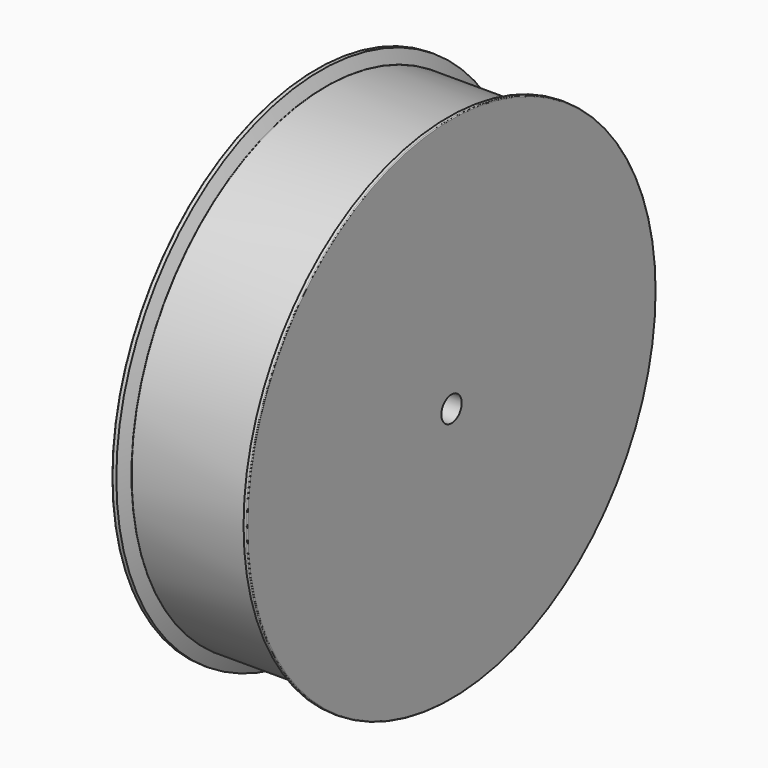
from build123d import *

# Parameters (mm, degrees)
F2_R     = 12.7
F3_DEPTH = 134.8161187441


# Not quite as in the source:
# - a feature names something its author has since deleted; it is built from what else it names


with BuildPart() as f1:
    # F0 (on Top) → F1 (revolve)
    with BuildSketch(Plane.XY):
        with BuildLine():
            Line((-3.6245174784, 29.0860664694), (-3.6245174784, 20.4818164694))
            Line((-3.6245174784, 20.4818164694), (-1.6004623353, 20.4818164694))
            ThreePointArc((-1.6004623353, 20.4818164694), (-1.0616469681, 20.2586318366), (-0.8384623353, 19.7198164694))
            Line((-0.8384623353, 19.7198164694), (-0.8384623353, -224.6888160382))
            Line((-0.8384623353, -224.6888160382), (131.1906012657, -224.6888160382))
            Line((131.1906012657, -224.6888160382), (131.1906012657, 29.3111839618))
            ThreePointArc((131.1906012657, 29.3111839618), (130.967416633, 29.8499993291), (130.4286012657, 30.0731839618))
            Line((130.4286012657, 30.0731839618), (127.6640418936, 30.0731839618))
            Line((127.6640418936, 30.0731839618), (123.3422697523, 17.6397553064))
            ThreePointArc((123.3422697523, 17.6397553064), (123.1973905872, 17.4466211557), (122.967395476, 17.3731839618))
            Line((122.967395476, 17.3731839618), (6.1083994667, 17.3731839618))
            ThreePointArc((6.1083994667, 17.3731839618), (5.8880446333, 17.4399778914), (5.7418610892, 17.6178768884))
            Line((5.7418610892, 17.6178768884), (0.6640418936, 29.8480664694))
            Line((0.6640418936, 29.8480664694), (-2.8625174784, 29.8480664694))
            ThreePointArc((-2.8625174784, 29.8480664694), (-3.4013328457, 29.6248818366), (-3.6245174784, 29.0860664694))
        make_face()
    revolve(axis=Axis((65.1760694652, -224.6888160382, 0), (1, 0, 0)))

    # F2 (on face) → F3 (cut, through all)
    with BuildSketch(Plane.YZ.offset(131.1906012657)):
        with Locations((-224.6888160382, 0)):
            Circle(F2_R)
    extrude(amount=-F3_DEPTH, mode=Mode.SUBTRACT)


solid = f1.part
